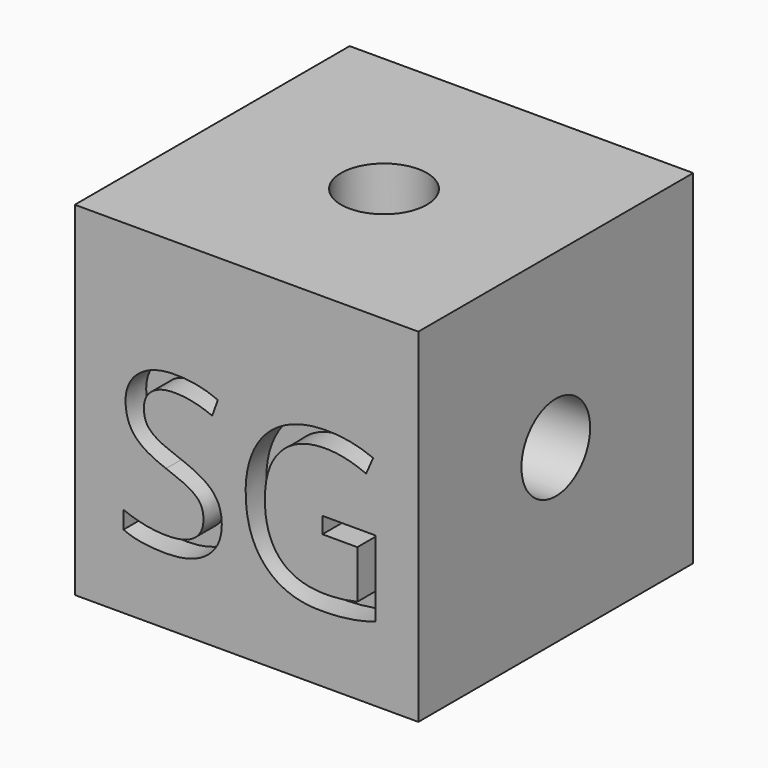
from build123d import *

# Parameters (mm, degrees)
F0_W         = 40
F0_H         = 40
F1_DEPTH     = 40
F2_TEXT_SIZE = 25.4651738538
F3_DEPTH     = 3
F4_R         = 5
F5_DEPTH     = 10
F6_R         = 5
F7_DEPTH     = 10
F8_R         = 5
F9_DEPTH     = 10
F10_R        = 5
F11_DEPTH    = 10


# Not quite as in the source:
# - Text() gives the source's letters only with a copy of the font that has no kerning and outlines rounded to 1/6400 em; it was checked with that copy


with BuildPart() as f1:
    # F0 (on Front) → F1 (new body)
    with BuildSketch(Plane.XZ):
        with Locations((20, 20)):
            Rectangle(F0_W, F0_H)
    extrude(amount=F1_DEPTH)

    # F2 (on face) → F3 (cut)
    with BuildSketch(Plane.XZ.offset(40)):
        with Locations((4.3583028018, 7.9651717097)):
            Text('SG', F2_TEXT_SIZE, font='Open Sans', text_align=(TextAlign.LEFT, TextAlign.BOTTOM))
    extrude(amount=-F3_DEPTH, mode=Mode.SUBTRACT)

    # F4 (on face) → F5 (cut)
    with BuildSketch(Plane(origin=(0, 0, 0), x_dir=(0, -1, 0), z_dir=(-1, 0, 0))):
        with Locations((20, 20)):
            Circle(F4_R)
    extrude(amount=-F5_DEPTH, mode=Mode.SUBTRACT)

    # F6 (on face) → F7 (cut)
    with BuildSketch(Plane.YZ.offset(40)):
        with Locations((-20, 20)):
            Circle(F6_R)
    extrude(amount=-F7_DEPTH, mode=Mode.SUBTRACT)

    # F8 (on face) → F9 (cut)
    with BuildSketch(Plane.XY.offset(40)):
        with Locations((20, -20)):
            Circle(F8_R)
    extrude(amount=-F9_DEPTH, mode=Mode.SUBTRACT)

    # F10 (on face) → F11 (cut)
    with BuildSketch(Plane(origin=(0, 0, 0), x_dir=(1, 0, 0), z_dir=(0, 0, -1))):
        with Locations((20, 20)):
            Circle(F10_R)
    extrude(amount=-F11_DEPTH, mode=Mode.SUBTRACT)


solid = f1.part
